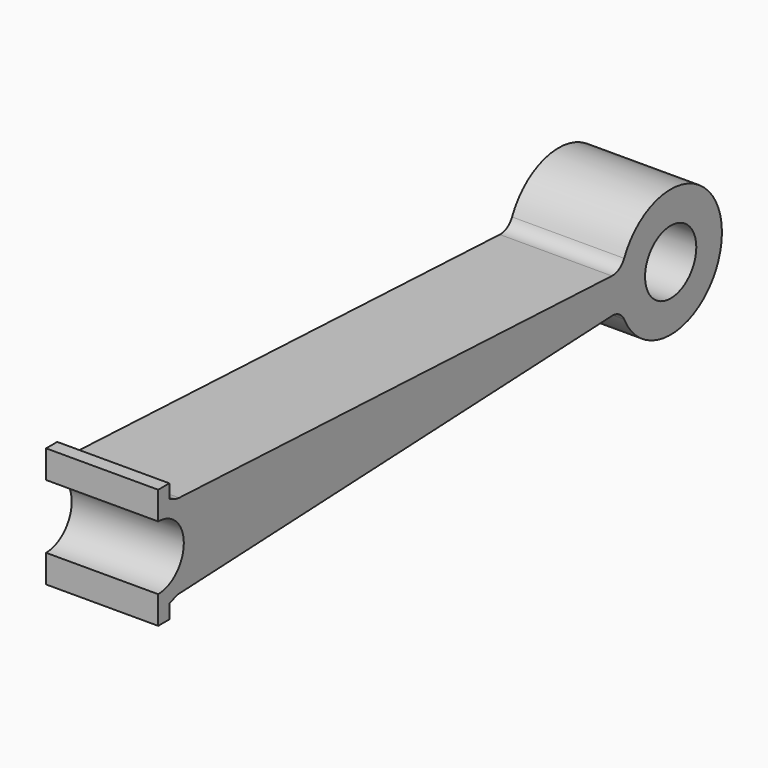
from build123d import *

# Parameters (mm, degrees)
F0_R     = 10
F1_DEPTH = 35
F2_R     = 5


# Not quite as in the source:
# - a feature names something its author has since deleted; it is built from what else it names


with BuildPart() as f1:
    # F0 (on Right) → F1 (new body)
    with BuildSketch(Plane.YZ):
        with BuildLine():
            Line((7.1040201683, -13.2110899417), (180.721386468, -5.3230686907))
            ThreePointArc((180.721386468, -5.3230686907), (220, 0), (180.721386468, 5.3230686907))
            Line((180.721386468, 5.3230686907), (7.1040201683, 13.2110899417))
            ThreePointArc((7.1040201683, 13.2110899417), (5.7575186768, 13.8510280733), (4.3541434669, 14.3541434669))
            Line((4.3541434669, 14.3541434669), (4.3541434669, 18.7082869339))
            Line((4.3541434669, 18.7082869339), (0, 18.7082869339))
            Line((0, 18.7082869339), (0, 14.3541434669))
            Line((0, 14.3541434669), (0, 10))
            ThreePointArc((0, 10), (10, 0), (0, -10))
            Line((0, -10), (0, -14.3541434669))
            Line((0, -14.3541434669), (0, -18.7082869339))
            Line((0, -18.7082869339), (4.3541434669, -18.7082869339))
            Line((4.3541434669, -18.7082869339), (4.3541434669, -14.3541434669))
            ThreePointArc((4.3541434669, -14.3541434669), (5.7575186768, -13.8510280733), (7.1040201683, -13.2110899417))
        make_face()
        with Locations((200, 0)):
            Circle(F0_R, mode=Mode.SUBTRACT)
    extrude(amount=F1_DEPTH)

    # F2
    f2_edges = [f1.edges().sort_by_distance(p)[0] for p in [
        (17.5, 7.10402, 13.21109),
        (17.5, 180.721386, 5.323069),
        (17.5, 180.721386, -5.323069),
        (17.5, 7.10402, -13.21109),
    ]]
    fillet(f2_edges, radius=F2_R)


solid = f1.part
